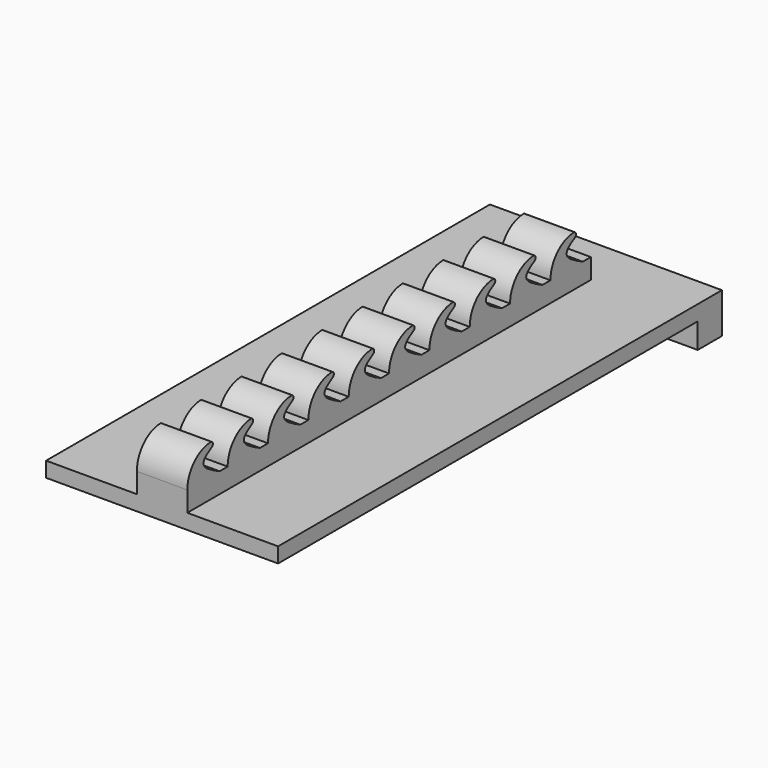
from build123d import *

# Parameters (mm, degrees)
F0_W     = 23
F0_H     = 52
F1_DEPTH = 1.5
F2_W     = 23
F2_H     = 4
F3_DEPTH = 3
F5_DEPTH = 2
F6_W     = 5
F6_H     = 4
F7_DEPTH = 3
F9_DEPTH = 5.1
F10_R    = 2.99999
F11_R    = 0.2684562318


# Not quite as in the source:
# - a fillet or chamfer is up to 0.001 mm smaller than in the source, because OpenCascade refuses the exact size


with BuildPart() as f1:
    # F0 (on Top) → F1 (new body)
    with BuildSketch(Plane.XY):
        with Locations((-1.6282885335, -0.8969272378)):
            Rectangle(F0_W, F0_H)
    extrude(amount=F1_DEPTH)

    # F2 (on face) → F3 (join)
    with BuildSketch(Plane(origin=(0, 25.1030727622, 0), x_dir=(-1, 0, 0), z_dir=(0, 1, 0))):
        with Locations((1.6282885335, -0.5)):
            Rectangle(F2_W, F2_H)
    extrude(amount=F3_DEPTH)

    # F4 (on face) → F5 (join)
    with BuildSketch(Plane.XY.offset(1.5)):
        Polygon((-4.1282885335, -26.8969272378), (-1.6282885335, -26.8969272378), (0, -26.8969272378), (0.8717114665, -26.8969272378), (0.8717114665, 23.1030727622), (-4.1282885335, 23.1030727622), align=None)
    extrude(amount=F5_DEPTH)

    # F6 (on face) → F7 (join)
    with BuildSketch(Plane.XY.offset(3.5)):
        with Locations((-1.6282885335, -24.8969272378)):
            Rectangle(F6_W, F6_H)
        with Locations((-1.6282885335, -19.8969272378)):
            Rectangle(F6_W, F6_H)
        with Locations((-1.6282885335, -14.8969272378)):
            Rectangle(F6_W, F6_H)
        with Locations((-1.6282885335, -9.8969272378)):
            Rectangle(F6_W, F6_H)
        with Locations((-1.6282885335, -4.8969272378)):
            Rectangle(F6_W, F6_H)
        with Locations((-1.6282885335, 0.1030727622)):
            Rectangle(F6_W, F6_H)
        with Locations((-1.6282885335, 5.1030727622)):
            Rectangle(F6_W, F6_H)
        with Locations((-1.6282885335, 10.1030727622)):
            Rectangle(F6_W, F6_H)
        with Locations((-1.6282885335, 15.1030727622)):
            Rectangle(F6_W, F6_H)
        with Locations((-1.6282885335, 20.1030727622)):
            Rectangle(F6_W, F6_H)
    extrude(amount=F7_DEPTH)

    # F8 (on face) → F9 (cut)
    with BuildSketch(Plane(origin=(-4.1282885335, 0, 0), x_dir=(0, -1, 0), z_dir=(-1, 0, 0))):
        with BuildLine():
            Line((22.8969272378, 6.5), (22.8969272378, 3.5))
            add(Edge.make_bspline(
                [(22.8969272378, 3.5), (23.8969272378, 4), (25.8969272378, 5), (23.8969272378, 6), (22.8969272378, 6.5)],
                knots=[0, 0, 0, 0, 0.5, 1, 1, 1, 1], degree=3))
        make_face()
        with BuildLine():
            Line((17.8969272378, 6.5), (17.8969272378, 3.5))
            add(Edge.make_bspline(
                [(17.8969272378, 3.5), (18.8969272378, 4), (20.8969272378, 5), (18.8969272378, 6), (17.8969272378, 6.5)],
                knots=[0, 0, 0, 0, 0.5, 1, 1, 1, 1], degree=3))
        make_face()
        with BuildLine():
            Line((12.8969272378, 6.5), (12.8969272378, 3.5))
            add(Edge.make_bspline(
                [(12.8969272378, 3.5), (13.8969272378, 4), (15.8969272378, 5), (13.8969272378, 6), (12.8969272378, 6.5)],
                knots=[0, 0, 0, 0, 0.5, 1, 1, 1, 1], degree=3))
        make_face()
        with BuildLine():
            Line((7.8969272378, 6.5), (7.8969272378, 3.5))
            add(Edge.make_bspline(
                [(7.8969272378, 3.5), (8.8969272378, 4), (10.8969272378, 5), (8.8969272378, 6), (7.8969272378, 6.5)],
                knots=[0, 0, 0, 0, 0.5, 1, 1, 1, 1], degree=3))
        make_face()
        with BuildLine():
            Line((2.8969272378, 6.5), (2.8969272378, 3.5))
            add(Edge.make_bspline(
                [(2.8969272378, 3.5), (3.8969272378, 4), (5.8969272378, 5), (3.8969272378, 6), (2.8969272378, 6.5)],
                knots=[0, 0, 0, 0, 0.5, 1, 1, 1, 1], degree=3))
        make_face()
        with BuildLine():
            Line((-2.1030727622, 6.5), (-2.1030727622, 3.5))
            add(Edge.make_bspline(
                [(-2.1030727622, 3.5), (-1.1030727622, 4), (0.8969272378, 5), (-1.1030727622, 6), (-2.1030727622, 6.5)],
                knots=[0, 0, 0, 0, 0.5, 1, 1, 1, 1], degree=3))
        make_face()
        with BuildLine():
            Line((-7.1030727622, 6.5), (-7.1030727622, 3.5))
            add(Edge.make_bspline(
                [(-7.1030727622, 3.5), (-6.1030727622, 4), (-4.1030727622, 5), (-6.1030727622, 6), (-7.1030727622, 6.5)],
                knots=[0, 0, 0, 0, 0.5, 1, 1, 1, 1], degree=3))
        make_face()
        with BuildLine():
            Line((-12.1030727622, 6.5), (-12.1030727622, 3.5))
            add(Edge.make_bspline(
                [(-12.1030727622, 3.5), (-11.1030727622, 4), (-9.1030727622, 5), (-11.1030727622, 6), (-12.1030727622, 6.5)],
                knots=[0, 0, 0, 0, 0.5, 1, 1, 1, 1], degree=3))
        make_face()
        with BuildLine():
            Line((-17.1030727622, 6.5), (-17.1030727622, 3.5))
            add(Edge.make_bspline(
                [(-17.1030727622, 3.5), (-16.1030727622, 4), (-14.1030727622, 5), (-16.1030727622, 6), (-17.1030727622, 6.5)],
                knots=[0, 0, 0, 0, 0.5, 1, 1, 1, 1], degree=3))
        make_face()
        with BuildLine():
            Line((-22.1030727622, 6.5), (-22.1030727622, 3.5))
            add(Edge.make_bspline(
                [(-22.1030727622, 3.5), (-21.1030727622, 4), (-19.1030727622, 5), (-21.1030727622, 6), (-22.1030727622, 6.5)],
                knots=[0, 0, 0, 0, 0.5, 1, 1, 1, 1], degree=3))
        make_face()
    extrude(amount=-F9_DEPTH, mode=Mode.SUBTRACT)

    # F10 (radius 3 in the source; OpenCascade refuses exactly that, so slightly less here)
    f10_edges = [f1.edges().sort_by_distance(p)[0] for p in [
        (-1.628289, -26.896927, 6.5),
        (-1.628289, -21.896927, 6.5),
        (-1.628289, -16.896927, 6.5),
        (-1.628289, -11.896927, 6.5),
        (-1.628289, -6.896927, 6.5),
        (-1.628289, -1.896927, 6.5),
        (-1.628289, 3.103073, 6.5),
        (-1.628289, 8.103073, 6.5),
        (-1.628289, 13.103073, 6.5),
        (-1.628289, 18.103073, 6.5),
    ]]
    fillet(f10_edges, radius=F10_R)

    # F11
    f11_edges = [f1.edges().sort_by_distance(p)[0] for p in [
        (-1.628289, -22.896927, 6.5),
        (-1.628289, 22.103073, 6.5),
        (-1.628289, 17.103073, 6.5),
        (-1.628289, 12.103073, 6.5),
        (-1.628289, 7.103073, 6.5),
        (-1.628289, -2.896927, 6.5),
        (-1.628289, -7.896927, 6.5),
        (-1.628289, -12.896927, 6.5),
        (-1.628289, -17.896927, 6.5),
        (-1.628289, 2.103073, 6.5),
    ]]
    fillet(f11_edges, radius=F11_R)


solid = f1.part
